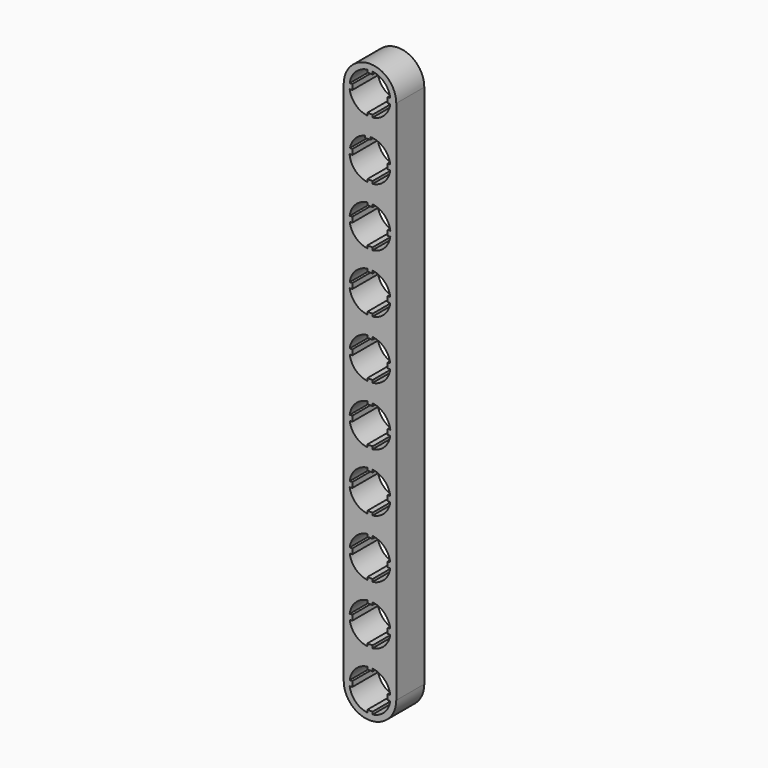
from build123d import *

# Parameters (mm, degrees)
F1_DEPTH = 7.62


# Not quite as in the source:
# - a feature names something its author has since deleted; it is built from what else it names


with BuildPart() as f1:
    # F0 (on Front) → F1 (new body)
    with BuildSketch(Plane.XZ):
        with BuildLine():
            ThreePointArc((-5.715, 47.4482442445), (0, 41.7332442445), (5.715, 47.4482442445))
            ThreePointArc((5.715, 47.4482442445), (0, 53.1632442445), (-5.715, 47.4482442445))
        make_face()
        with BuildLine():
            ThreePointArc((4.4081076155, 48.0197442445), (4.4357673153, 47.7345890096), (4.445, 47.4482442445))
            ThreePointArc((4.445, 47.4482442445), (4.4357673153, 47.1618994794), (4.4081076155, 46.8767442445))
            ThreePointArc((4.4081076155, 46.8767442445), (3.1430896424, 44.3051546021), (0.5715, 43.040136629))
            ThreePointArc((0.5715, 43.040136629), (0, 43.0032442445), (-0.5715, 43.040136629))
            ThreePointArc((-0.5715, 43.040136629), (-3.1430896424, 44.3051546021), (-4.4081076155, 46.8767442445))
            ThreePointArc((-4.4081076155, 46.8767442445), (-4.445, 47.4482442445), (-4.4081076155, 48.0197442445))
            ThreePointArc((-4.4081076155, 48.0197442445), (-3.1430896424, 50.5913338869), (-0.5715, 51.85635186))
            ThreePointArc((-0.5715, 51.85635186), (0, 51.8932442445), (0.5715, 51.85635186))
            ThreePointArc((0.5715, 51.85635186), (3.1430896424, 50.5913338869), (4.4081076155, 48.0197442445))
        make_face(mode=Mode.SUBTRACT)
        with BuildLine():
            Line((5.715, 34.7482442445), (5.715, 47.4482442445))
            ThreePointArc((5.715, 47.4482442445), (0, 41.7332442445), (-5.715, 47.4482442445))
            Line((-5.715, 47.4482442445), (-5.715, 34.7482442445))
            ThreePointArc((-5.715, 34.7482442445), (0, 40.4632442445), (5.715, 34.7482442445))
        make_face()
        with BuildLine():
            ThreePointArc((-5.715, 34.7482442445), (0, 29.0332442445), (5.715, 34.7482442445))
            ThreePointArc((5.715, 34.7482442445), (0, 40.4632442445), (-5.715, 34.7482442445))
        make_face()
        with BuildLine():
            ThreePointArc((4.4081076155, 35.3197442445), (4.4357673153, 35.0345890096), (4.445, 34.7482442445))
            ThreePointArc((4.445, 34.7482442445), (4.4357673153, 34.4618994794), (4.4081076155, 34.1767442445))
            ThreePointArc((4.4081076155, 34.1767442445), (3.1430896424, 31.6051546021), (0.5715, 30.340136629))
            ThreePointArc((0.5715, 30.340136629), (0, 30.3032442445), (-0.5715, 30.340136629))
            ThreePointArc((-0.5715, 30.340136629), (-3.2458434243, 31.7113831241), (-4.4363415477, 34.4709381461))
            ThreePointArc((-4.4363415477, 34.4709381461), (-4.4350889005, 35.0449114731), (-4.3598852128, 35.6139381461))
            ThreePointArc((-4.3598852128, 35.6139381461), (-3.2117417195, 37.821148429), (-1.0573885644, 39.0656455953))
            ThreePointArc((-1.0573885644, 39.0656455953), (-0.4900057315, 39.1661531823), (0.0856114356, 39.1924197228))
            ThreePointArc((0.0856114356, 39.1924197228), (2.9661054546, 38.0588700814), (4.4081076155, 35.3197442445))
        make_face(mode=Mode.SUBTRACT)
        with BuildLine():
            Line((5.715, 22.0482442445), (5.715, 34.7482442445))
            ThreePointArc((5.715, 34.7482442445), (0, 29.0332442445), (-5.715, 34.7482442445))
            Line((-5.715, 34.7482442445), (-5.715, 22.0482442445))
            ThreePointArc((-5.715, 22.0482442445), (0, 27.7632442445), (5.715, 22.0482442445))
        make_face()
        with BuildLine():
            ThreePointArc((-5.715, 22.0482442445), (0, 16.3332442445), (5.715, 22.0482442445))
            ThreePointArc((5.715, 22.0482442445), (0, 27.7632442445), (-5.715, 22.0482442445))
        make_face()
        with BuildLine():
            ThreePointArc((4.4081076155, 22.6197442445), (4.4357673153, 22.3345890096), (4.445, 22.0482442445))
            ThreePointArc((4.445, 22.0482442445), (4.4357673153, 21.7618994794), (4.4081076155, 21.4767442445))
            ThreePointArc((4.4081076155, 21.4767442445), (3.1430896424, 18.9051546021), (0.5715, 17.640136629))
            ThreePointArc((0.5715, 17.640136629), (0, 17.6032442445), (-0.5715, 17.640136629))
            ThreePointArc((-0.5715, 17.640136629), (-3.1430896424, 18.9051546021), (-4.4081076155, 21.4767442445))
            ThreePointArc((-4.4081076155, 21.4767442445), (-4.445, 22.0482442445), (-4.4081076155, 22.6197442445))
            ThreePointArc((-4.4081076155, 22.6197442445), (-3.1430896424, 25.1913338869), (-0.5715, 26.45635186))
            ThreePointArc((-0.5715, 26.45635186), (0, 26.4932442445), (0.5715, 26.45635186))
            ThreePointArc((0.5715, 26.45635186), (3.1430896424, 25.1913338869), (4.4081076155, 22.6197442445))
        make_face(mode=Mode.SUBTRACT)
        with BuildLine():
            Line((5.715, 9.3482442445), (5.715, 22.0482442445))
            ThreePointArc((5.715, 22.0482442445), (0, 16.3332442445), (-5.715, 22.0482442445))
            Line((-5.715, 22.0482442445), (-5.715, 9.348244273))
            ThreePointArc((-5.715, 9.348244273), (1.42e-08, 15.0632442445), (5.715, 9.3482442445))
        make_face()
        with BuildLine():
            ThreePointArc((-5.715, 9.348244273), (-1.42e-08, 3.6332442445), (5.715, 9.3482442445))
            ThreePointArc((5.715, 9.3482442445), (1.42e-08, 15.0632442445), (-5.715, 9.348244273))
        make_face()
        with BuildLine():
            ThreePointArc((4.4081076155, 9.9197442445), (4.4357673153, 9.6345890096), (4.445, 9.3482442445))
            ThreePointArc((4.445, 9.3482442445), (4.4357673153, 9.0618994794), (4.4081076155, 8.7767442445))
            ThreePointArc((4.4081076155, 8.7767442445), (3.1430896424, 6.2051546021), (0.5715, 4.940136629))
            ThreePointArc((0.5715, 4.940136629), (0, 4.9032442445), (-0.5715, 4.940136629))
            ThreePointArc((-0.5715, 4.940136629), (-3.1430896424, 6.2051546021), (-4.4081076155, 8.7767442445))
            ThreePointArc((-4.4081076155, 8.7767442445), (-4.445, 9.3482442445), (-4.4081076155, 9.9197442445))
            ThreePointArc((-4.4081076155, 9.9197442445), (-3.1430896424, 12.4913338869), (-0.5715, 13.75635186))
            ThreePointArc((-0.5715, 13.75635186), (0, 13.7932442445), (0.5715, 13.75635186))
            ThreePointArc((0.5715, 13.75635186), (3.1430896424, 12.4913338869), (4.4081076155, 9.9197442445))
        make_face(mode=Mode.SUBTRACT)
        with BuildLine():
            Line((5.715, -3.3517557555), (5.715, 9.3482442445))
            ThreePointArc((5.715, 9.3482442445), (-1.42e-08, 3.6332442445), (-5.715, 9.348244273))
            Line((-5.715, 9.348244273), (-5.715, -3.3517557536))
            ThreePointArc((-5.715, -3.3517557536), (9e-10, 2.3632442445), (5.715, -3.3517557555))
        make_face()
        with BuildLine():
            ThreePointArc((-5.715, -3.3517557536), (-9e-10, -9.0667557555), (5.715, -3.3517557555))
            ThreePointArc((5.715, -3.3517557555), (9e-10, 2.3632442445), (-5.715, -3.3517557536))
        make_face()
        with BuildLine():
            ThreePointArc((4.4081076155, -2.7802557555), (4.4357673153, -3.0654109904), (4.445, -3.3517557555))
            ThreePointArc((4.445, -3.3517557555), (4.4357673153, -3.6381005206), (4.4081076155, -3.9232557555))
            ThreePointArc((4.4081076155, -3.9232557555), (3.1430896424, -6.4948453979), (0.5715, -7.759863371))
            ThreePointArc((0.5715, -7.759863371), (0, -7.7967557555), (-0.5715, -7.759863371))
            ThreePointArc((-0.5715, -7.759863371), (-3.1430896424, -6.4948453979), (-4.4081076155, -3.9232557555))
            ThreePointArc((-4.4081076155, -3.9232557555), (-4.445, -3.3517557555), (-4.4081076155, -2.7802557555))
            ThreePointArc((-4.4081076155, -2.7802557555), (-3.1430896424, -0.2086661131), (-0.5715, 1.05635186))
            ThreePointArc((-0.5715, 1.05635186), (0, 1.0932442445), (0.5715, 1.05635186))
            ThreePointArc((0.5715, 1.05635186), (3.1430896424, -0.2086661131), (4.4081076155, -2.7802557555))
        make_face(mode=Mode.SUBTRACT)
        with BuildLine():
            Line((5.715, -16.0517557555), (5.715, -3.3517557555))
            ThreePointArc((5.715, -3.3517557555), (-9e-10, -9.0667557555), (-5.715, -3.3517557536))
            Line((-5.715, -3.3517557536), (-5.715, -16.0517557555))
            ThreePointArc((-5.715, -16.0517557555), (0, -10.3367557555), (5.715, -16.0517557555))
        make_face()
        with BuildLine():
            ThreePointArc((-5.715, -16.0517557555), (0, -21.7667557555), (5.715, -16.0517557555))
            ThreePointArc((5.715, -16.0517557555), (0, -10.3367557555), (-5.715, -16.0517557555))
        make_face()
        with BuildLine():
            ThreePointArc((4.4081076155, -15.4802557555), (4.4357673153, -15.7654109904), (4.445, -16.0517557555))
            ThreePointArc((4.445, -16.0517557555), (4.4357673153, -16.3381005206), (4.4081076155, -16.6232557555))
            ThreePointArc((4.4081076155, -16.6232557555), (3.1430896424, -19.1948453979), (0.5715, -20.459863371))
            ThreePointArc((0.5715, -20.459863371), (0, -20.4967557555), (-0.5715, -20.459863371))
            ThreePointArc((-0.5715, -20.459863371), (-3.1430896424, -19.1948453979), (-4.4081076155, -16.6232557555))
            ThreePointArc((-4.4081076155, -16.6232557555), (-4.445, -16.0517557555), (-4.4081076155, -15.4802557555))
            ThreePointArc((-4.4081076155, -15.4802557555), (-3.1430896424, -12.9086661131), (-0.5715, -11.64364814))
            ThreePointArc((-0.5715, -11.64364814), (0, -11.6067557555), (0.5715, -11.64364814))
            ThreePointArc((0.5715, -11.64364814), (3.1430896424, -12.9086661131), (4.4081076155, -15.4802557555))
        make_face(mode=Mode.SUBTRACT)
        with BuildLine():
            Line((5.715, -28.7517557555), (5.715, -16.0517557555))
            ThreePointArc((5.715, -16.0517557555), (0, -21.7667557555), (-5.715, -16.0517557555))
            Line((-5.715, -16.0517557555), (-5.715, -28.7517557555))
            ThreePointArc((-5.715, -28.7517557555), (0, -23.0367557555), (5.715, -28.7517557555))
        make_face()
        with BuildLine():
            ThreePointArc((-5.715, -28.7517557555), (0, -34.4667557555), (5.715, -28.7517557555))
            ThreePointArc((5.715, -28.7517557555), (0, -23.0367557555), (-5.715, -28.7517557555))
        make_face()
        with BuildLine():
            ThreePointArc((4.4081076155, -28.1802557555), (4.4357673153, -28.4654109904), (4.445, -28.7517557555))
            ThreePointArc((4.445, -28.7517557555), (4.4357673153, -29.0381005206), (4.4081076155, -29.3232557555))
            ThreePointArc((4.4081076155, -29.3232557555), (3.1430896424, -31.8948453979), (0.5715, -33.159863371))
            ThreePointArc((0.5715, -33.159863371), (0, -33.1967557555), (-0.5715, -33.159863371))
            ThreePointArc((-0.5715, -33.159863371), (-3.1430896424, -31.8948453979), (-4.4081076155, -29.3232557555))
            ThreePointArc((-4.4081076155, -29.3232557555), (-4.445, -28.7517557555), (-4.4081076155, -28.1802557555))
            ThreePointArc((-4.4081076155, -28.1802557555), (-3.1430896424, -25.6086661131), (-0.5715, -24.34364814))
            ThreePointArc((-0.5715, -24.34364814), (0, -24.3067557555), (0.5715, -24.34364814))
            ThreePointArc((0.5715, -24.34364814), (3.1430896424, -25.6086661131), (4.4081076155, -28.1802557555))
        make_face(mode=Mode.SUBTRACT)
        with BuildLine():
            Line((5.715, -41.4517557555), (5.715, -28.7517557555))
            ThreePointArc((5.715, -28.7517557555), (0, -34.4667557555), (-5.715, -28.7517557555))
            Line((-5.715, -28.7517557555), (-5.715, -41.4517557757))
            ThreePointArc((-5.715, -41.4517557757), (-1.01e-08, -35.7367557555), (5.715, -41.4517557555))
        make_face()
        with BuildLine():
            ThreePointArc((-5.715, -41.4517557757), (1.01e-08, -47.1667557555), (5.715, -41.4517557555))
            ThreePointArc((5.715, -41.4517557555), (-1.01e-08, -35.7367557555), (-5.715, -41.4517557757))
        make_face()
        with BuildLine():
            ThreePointArc((4.4081076155, -40.8802557555), (4.4357673153, -41.1654109904), (4.445, -41.4517557555))
            ThreePointArc((4.445, -41.4517557555), (4.4357673153, -41.7381005206), (4.4081076155, -42.0232557555))
            ThreePointArc((4.4081076155, -42.0232557555), (3.1430896424, -44.5948453979), (0.5715, -45.859863371))
            ThreePointArc((0.5715, -45.859863371), (0, -45.8967557555), (-0.5715, -45.859863371))
            ThreePointArc((-0.5715, -45.859863371), (-3.1430896424, -44.5948453979), (-4.4081076155, -42.0232557555))
            ThreePointArc((-4.4081076155, -42.0232557555), (-4.445, -41.4517557555), (-4.4081076155, -40.8802557555))
            ThreePointArc((-4.4081076155, -40.8802557555), (-3.1430896424, -38.3086661131), (-0.5715, -37.04364814))
            ThreePointArc((-0.5715, -37.04364814), (0, -37.0067557555), (0.5715, -37.04364814))
            ThreePointArc((0.5715, -37.04364814), (3.1430896424, -38.3086661131), (4.4081076155, -40.8802557555))
        make_face(mode=Mode.SUBTRACT)
        with BuildLine():
            Line((5.715, -54.1517557555), (5.715, -41.4517557555))
            ThreePointArc((5.715, -41.4517557555), (1.01e-08, -47.1667557555), (-5.715, -41.4517557757))
            Line((-5.715, -41.4517557757), (-5.715, -54.1517557757))
            ThreePointArc((-5.715, -54.1517557757), (-1.01e-08, -48.4367557555), (5.715, -54.1517557555))
        make_face()
        with BuildLine():
            ThreePointArc((-5.715, -54.1517557757), (1.01e-08, -59.8667557555), (5.715, -54.1517557555))
            ThreePointArc((5.715, -54.1517557555), (-1.01e-08, -48.4367557555), (-5.715, -54.1517557757))
        make_face()
        with BuildLine():
            ThreePointArc((4.4081076155, -53.5802557555), (4.4357673153, -53.8654109904), (4.445, -54.1517557555))
            ThreePointArc((4.445, -54.1517557555), (4.4357673153, -54.4381005206), (4.4081076155, -54.7232557555))
            ThreePointArc((4.4081076155, -54.7232557555), (3.1430896424, -57.2948453979), (0.5715, -58.559863371))
            ThreePointArc((0.5715, -58.559863371), (0, -58.5967557555), (-0.5715, -58.559863371))
            ThreePointArc((-0.5715, -58.559863371), (-3.1430896424, -57.2948453979), (-4.4081076155, -54.7232557555))
            ThreePointArc((-4.4081076155, -54.7232557555), (-4.445, -54.1517557555), (-4.4081076155, -53.5802557555))
            ThreePointArc((-4.4081076155, -53.5802557555), (-3.1430896424, -51.0086661131), (-0.5715, -49.74364814))
            ThreePointArc((-0.5715, -49.74364814), (0, -49.7067557555), (0.5715, -49.74364814))
            ThreePointArc((0.5715, -49.74364814), (3.1430896424, -51.0086661131), (4.4081076155, -53.5802557555))
        make_face(mode=Mode.SUBTRACT)
        with BuildLine():
            Line((5.715, -66.8517557555), (5.715, -54.1517557555))
            ThreePointArc((5.715, -54.1517557555), (1.01e-08, -59.8667557555), (-5.715, -54.1517557757))
            Line((-5.715, -54.1517557757), (-5.715, -66.8517557555))
            ThreePointArc((-5.715, -66.8517557555), (0, -61.1367557555), (5.715, -66.8517557555))
        make_face()
        with BuildLine():
            ThreePointArc((-5.715, -66.8517557555), (0, -72.5667557555), (5.715, -66.8517557555))
            ThreePointArc((5.715, -66.8517557555), (0, -61.1367557555), (-5.715, -66.8517557555))
        make_face()
        with BuildLine():
            ThreePointArc((4.4081076155, -66.2802557555), (4.4357673153, -66.5654109904), (4.445, -66.8517557555))
            ThreePointArc((4.445, -66.8517557555), (4.4357673153, -67.1381005206), (4.4081076155, -67.4232557555))
            ThreePointArc((4.4081076155, -67.4232557555), (3.1430896424, -69.9948453979), (0.5715, -71.259863371))
            ThreePointArc((0.5715, -71.259863371), (0, -71.2967557555), (-0.5715, -71.259863371))
            ThreePointArc((-0.5715, -71.259863371), (-3.1430896424, -69.9948453979), (-4.4081076155, -67.4232557555))
            ThreePointArc((-4.4081076155, -67.4232557555), (-4.445, -66.8517557555), (-4.4081076155, -66.2802557555))
            ThreePointArc((-4.4081076155, -66.2802557555), (-3.1430896424, -63.7086661131), (-0.5715, -62.44364814))
            ThreePointArc((-0.5715, -62.44364814), (0, -62.4067557555), (0.5715, -62.44364814))
            ThreePointArc((0.5715, -62.44364814), (3.1430896424, -63.7086661131), (4.4081076155, -66.2802557555))
        make_face(mode=Mode.SUBTRACT)
        with BuildLine():
            Line((0.5715, 51.29755186), (0.5715, 51.85635186))
            ThreePointArc((0.5715, 51.85635186), (0, 51.8932442445), (-0.5715, 51.85635186))
            Line((-0.5715, 51.85635186), (-0.5715, 51.29755186))
            Line((-0.5715, 51.29755186), (0.5715, 51.29755186))
        make_face()
        with BuildLine():
            ThreePointArc((4.4081076155, 46.8767442445), (4.4357673153, 47.1618994794), (4.445, 47.4482442445))
            ThreePointArc((4.445, 47.4482442445), (4.4357673153, 47.7345890096), (4.4081076155, 48.0197442445))
            Line((4.4081076155, 48.0197442445), (3.8493076155, 48.0197442445))
            Line((3.8493076155, 48.0197442445), (3.8493076155, 46.8767442445))
            Line((3.8493076155, 46.8767442445), (4.4081076155, 46.8767442445))
        make_face()
        with BuildLine():
            ThreePointArc((-0.5715, 43.040136629), (0, 43.0032442445), (0.5715, 43.040136629))
            Line((0.5715, 43.040136629), (0.5715, 43.598936629))
            Line((0.5715, 43.598936629), (-0.5715, 43.598936629))
            Line((-0.5715, 43.598936629), (-0.5715, 43.040136629))
        make_face()
        with BuildLine():
            Line((-3.8493076155, 48.0197442445), (-4.4081076155, 48.0197442445))
            ThreePointArc((-4.4081076155, 48.0197442445), (-4.445, 47.4482442445), (-4.4081076155, 46.8767442445))
            Line((-4.4081076155, 46.8767442445), (-3.8493076155, 46.8767442445))
            Line((-3.8493076155, 46.8767442445), (-3.8493076155, 48.0197442445))
        make_face()
        with BuildLine():
            ThreePointArc((4.4081076155, -67.4232557555), (4.4357673153, -67.1381005206), (4.445, -66.8517557555))
            ThreePointArc((4.445, -66.8517557555), (4.4357673153, -66.5654109904), (4.4081076155, -66.2802557555))
            Line((4.4081076155, -66.2802557555), (3.8493076155, -66.2802557555))
            Line((3.8493076155, -66.2802557555), (3.8493076155, -67.4232557555))
            Line((3.8493076155, -67.4232557555), (4.4081076155, -67.4232557555))
        make_face()
        with BuildLine():
            ThreePointArc((4.4081076155, 8.7767442445), (4.4357673153, 9.0618994794), (4.445, 9.3482442445))
            ThreePointArc((4.445, 9.3482442445), (4.4357673153, 9.6345890096), (4.4081076155, 9.9197442445))
            Line((4.4081076155, 9.9197442445), (3.8493076155, 9.9197442445))
            Line((3.8493076155, 9.9197442445), (3.8493076155, 8.7767442445))
            Line((3.8493076155, 8.7767442445), (4.4081076155, 8.7767442445))
        make_face()
        with BuildLine():
            Line((-3.8493076155, -15.4802557555), (-4.4081076155, -15.4802557555))
            ThreePointArc((-4.4081076155, -15.4802557555), (-4.445, -16.0517557555), (-4.4081076155, -16.6232557555))
            Line((-4.4081076155, -16.6232557555), (-3.8493076155, -16.6232557555))
            Line((-3.8493076155, -16.6232557555), (-3.8493076155, -15.4802557555))
        make_face()
        with BuildLine():
            Line((0.0856114356, 38.6336197228), (0.0856114356, 39.1924197228))
            ThreePointArc((0.0856114356, 39.1924197228), (-0.4900057315, 39.1661531823), (-1.0573885644, 39.0656455953))
            Line((-1.0573885644, 39.0656455953), (-1.0573885644, 38.6336197228))
            Line((-1.0573885644, 38.6336197228), (0.0856114356, 38.6336197228))
        make_face()
        with BuildLine():
            Line((-3.8010852128, 35.6139381461), (-4.3598852128, 35.6139381461))
            ThreePointArc((-4.3598852128, 35.6139381461), (-4.4350889005, 35.0449114731), (-4.4363415477, 34.4709381461))
            Line((-4.4363415477, 34.4709381461), (-3.8010852128, 34.4709381461))
            Line((-3.8010852128, 34.4709381461), (-3.8010852128, 35.6139381461))
        make_face()
        with BuildLine():
            ThreePointArc((-0.5715, 30.340136629), (0, 30.3032442445), (0.5715, 30.340136629))
            Line((0.5715, 30.340136629), (0.5715, 30.898936629))
            Line((0.5715, 30.898936629), (-0.5715, 30.898936629))
            Line((-0.5715, 30.898936629), (-0.5715, 30.340136629))
        make_face()
        with BuildLine():
            ThreePointArc((4.4081076155, 34.1767442445), (4.4357673153, 34.4618994794), (4.445, 34.7482442445))
            ThreePointArc((4.445, 34.7482442445), (4.4357673153, 35.0345890096), (4.4081076155, 35.3197442445))
            Line((4.4081076155, 35.3197442445), (3.8493076155, 35.3197442445))
            Line((3.8493076155, 35.3197442445), (3.8493076155, 34.1767442445))
            Line((3.8493076155, 34.1767442445), (4.4081076155, 34.1767442445))
        make_face()
        with BuildLine():
            Line((0.5715, 25.89755186), (0.5715, 26.45635186))
            ThreePointArc((0.5715, 26.45635186), (0, 26.4932442445), (-0.5715, 26.45635186))
            Line((-0.5715, 26.45635186), (-0.5715, 25.89755186))
            Line((-0.5715, 25.89755186), (0.5715, 25.89755186))
        make_face()
        with BuildLine():
            Line((-3.8493076155, 22.6197442445), (-4.4081076155, 22.6197442445))
            ThreePointArc((-4.4081076155, 22.6197442445), (-4.445, 22.0482442445), (-4.4081076155, 21.4767442445))
            Line((-4.4081076155, 21.4767442445), (-3.8493076155, 21.4767442445))
            Line((-3.8493076155, 21.4767442445), (-3.8493076155, 22.6197442445))
        make_face()
        with BuildLine():
            ThreePointArc((4.4081076155, 21.4767442445), (4.4357673153, 21.7618994794), (4.445, 22.0482442445))
            ThreePointArc((4.445, 22.0482442445), (4.4357673153, 22.3345890096), (4.4081076155, 22.6197442445))
            Line((4.4081076155, 22.6197442445), (3.8493076155, 22.6197442445))
            Line((3.8493076155, 22.6197442445), (3.8493076155, 21.4767442445))
            Line((3.8493076155, 21.4767442445), (4.4081076155, 21.4767442445))
        make_face()
        with BuildLine():
            ThreePointArc((-0.5715, 17.640136629), (0, 17.6032442445), (0.5715, 17.640136629))
            Line((0.5715, 17.640136629), (0.5715, 18.198936629))
            Line((0.5715, 18.198936629), (-0.5715, 18.198936629))
            Line((-0.5715, 18.198936629), (-0.5715, 17.640136629))
        make_face()
        with BuildLine():
            Line((0.5715, 13.19755186), (0.5715, 13.75635186))
            ThreePointArc((0.5715, 13.75635186), (0, 13.7932442445), (-0.5715, 13.75635186))
            Line((-0.5715, 13.75635186), (-0.5715, 13.19755186))
            Line((-0.5715, 13.19755186), (0.5715, 13.19755186))
        make_face()
        with BuildLine():
            Line((-3.8493076155, 9.9197442445), (-4.4081076155, 9.9197442445))
            ThreePointArc((-4.4081076155, 9.9197442445), (-4.445, 9.3482442445), (-4.4081076155, 8.7767442445))
            Line((-4.4081076155, 8.7767442445), (-3.8493076155, 8.7767442445))
            Line((-3.8493076155, 8.7767442445), (-3.8493076155, 9.9197442445))
        make_face()
        with BuildLine():
            ThreePointArc((-0.5715, 4.940136629), (0, 4.9032442445), (0.5715, 4.940136629))
            Line((0.5715, 4.940136629), (0.5715, 5.498936629))
            Line((0.5715, 5.498936629), (-0.5715, 5.498936629))
            Line((-0.5715, 5.498936629), (-0.5715, 4.940136629))
        make_face()
        with BuildLine():
            Line((0.5715, 0.49755186), (0.5715, 1.05635186))
            ThreePointArc((0.5715, 1.05635186), (0, 1.0932442445), (-0.5715, 1.05635186))
            Line((-0.5715, 1.05635186), (-0.5715, 0.49755186))
            Line((-0.5715, 0.49755186), (0.5715, 0.49755186))
        make_face()
        with BuildLine():
            ThreePointArc((4.4081076155, -3.9232557555), (4.4357673153, -3.6381005206), (4.445, -3.3517557555))
            ThreePointArc((4.445, -3.3517557555), (4.4357673153, -3.0654109904), (4.4081076155, -2.7802557555))
            Line((4.4081076155, -2.7802557555), (3.8493076155, -2.7802557555))
            Line((3.8493076155, -2.7802557555), (3.8493076155, -3.9232557555))
            Line((3.8493076155, -3.9232557555), (4.4081076155, -3.9232557555))
        make_face()
        with BuildLine():
            ThreePointArc((-0.5715, -7.759863371), (0, -7.7967557555), (0.5715, -7.759863371))
            Line((0.5715, -7.759863371), (0.5715, -7.201063371))
            Line((0.5715, -7.201063371), (-0.5715, -7.201063371))
            Line((-0.5715, -7.201063371), (-0.5715, -7.759863371))
        make_face()
        with BuildLine():
            Line((-3.8493076155, -2.7802557555), (-4.4081076155, -2.7802557555))
            ThreePointArc((-4.4081076155, -2.7802557555), (-4.445, -3.3517557555), (-4.4081076155, -3.9232557555))
            Line((-4.4081076155, -3.9232557555), (-3.8493076155, -3.9232557555))
            Line((-3.8493076155, -3.9232557555), (-3.8493076155, -2.7802557555))
        make_face()
        with BuildLine():
            Line((0.5715, -12.20244814), (0.5715, -11.64364814))
            ThreePointArc((0.5715, -11.64364814), (0, -11.6067557555), (-0.5715, -11.64364814))
            Line((-0.5715, -11.64364814), (-0.5715, -12.20244814))
            Line((-0.5715, -12.20244814), (0.5715, -12.20244814))
        make_face()
        with BuildLine():
            ThreePointArc((4.4081076155, -16.6232557555), (4.4357673153, -16.3381005206), (4.445, -16.0517557555))
            ThreePointArc((4.445, -16.0517557555), (4.4357673153, -15.7654109904), (4.4081076155, -15.4802557555))
            Line((4.4081076155, -15.4802557555), (3.8493076155, -15.4802557555))
            Line((3.8493076155, -15.4802557555), (3.8493076155, -16.6232557555))
            Line((3.8493076155, -16.6232557555), (4.4081076155, -16.6232557555))
        make_face()
        with BuildLine():
            ThreePointArc((-0.5715, -20.459863371), (0, -20.4967557555), (0.5715, -20.459863371))
            Line((0.5715, -20.459863371), (0.5715, -19.901063371))
            Line((0.5715, -19.901063371), (-0.5715, -19.901063371))
            Line((-0.5715, -19.901063371), (-0.5715, -20.459863371))
        make_face()
        with BuildLine():
            Line((0.5715, -24.90244814), (0.5715, -24.34364814))
            ThreePointArc((0.5715, -24.34364814), (0, -24.3067557555), (-0.5715, -24.34364814))
            Line((-0.5715, -24.34364814), (-0.5715, -24.90244814))
            Line((-0.5715, -24.90244814), (0.5715, -24.90244814))
        make_face()
        with BuildLine():
            ThreePointArc((4.4081076155, -29.3232557555), (4.4357673153, -29.0381005206), (4.445, -28.7517557555))
            ThreePointArc((4.445, -28.7517557555), (4.4357673153, -28.4654109904), (4.4081076155, -28.1802557555))
            Line((4.4081076155, -28.1802557555), (3.8493076155, -28.1802557555))
            Line((3.8493076155, -28.1802557555), (3.8493076155, -29.3232557555))
            Line((3.8493076155, -29.3232557555), (4.4081076155, -29.3232557555))
        make_face()
        with BuildLine():
            Line((-3.8493076155, -28.1802557555), (-4.4081076155, -28.1802557555))
            ThreePointArc((-4.4081076155, -28.1802557555), (-4.445, -28.7517557555), (-4.4081076155, -29.3232557555))
            Line((-4.4081076155, -29.3232557555), (-3.8493076155, -29.3232557555))
            Line((-3.8493076155, -29.3232557555), (-3.8493076155, -28.1802557555))
        make_face()
        with BuildLine():
            ThreePointArc((-0.5715, -33.159863371), (0, -33.1967557555), (0.5715, -33.159863371))
            Line((0.5715, -33.159863371), (0.5715, -32.601063371))
            Line((0.5715, -32.601063371), (-0.5715, -32.601063371))
            Line((-0.5715, -32.601063371), (-0.5715, -33.159863371))
        make_face()
        with BuildLine():
            Line((0.5715, -37.60244814), (0.5715, -37.04364814))
            ThreePointArc((0.5715, -37.04364814), (0, -37.0067557555), (-0.5715, -37.04364814))
            Line((-0.5715, -37.04364814), (-0.5715, -37.60244814))
            Line((-0.5715, -37.60244814), (0.5715, -37.60244814))
        make_face()
        with BuildLine():
            ThreePointArc((4.4081076155, -42.0232557555), (4.4357673153, -41.7381005206), (4.445, -41.4517557555))
            ThreePointArc((4.445, -41.4517557555), (4.4357673153, -41.1654109904), (4.4081076155, -40.8802557555))
            Line((4.4081076155, -40.8802557555), (3.8493076155, -40.8802557555))
            Line((3.8493076155, -40.8802557555), (3.8493076155, -42.0232557555))
            Line((3.8493076155, -42.0232557555), (4.4081076155, -42.0232557555))
        make_face()
        with BuildLine():
            Line((-3.8493076155, -40.8802557555), (-4.4081076155, -40.8802557555))
            ThreePointArc((-4.4081076155, -40.8802557555), (-4.445, -41.4517557555), (-4.4081076155, -42.0232557555))
            Line((-4.4081076155, -42.0232557555), (-3.8493076155, -42.0232557555))
            Line((-3.8493076155, -42.0232557555), (-3.8493076155, -40.8802557555))
        make_face()
        with BuildLine():
            ThreePointArc((-0.5715, -45.859863371), (0, -45.8967557555), (0.5715, -45.859863371))
            Line((0.5715, -45.859863371), (0.5715, -45.301063371))
            Line((0.5715, -45.301063371), (-0.5715, -45.301063371))
            Line((-0.5715, -45.301063371), (-0.5715, -45.859863371))
        make_face()
        with BuildLine():
            Line((0.5715, -50.30244814), (0.5715, -49.74364814))
            ThreePointArc((0.5715, -49.74364814), (0, -49.7067557555), (-0.5715, -49.74364814))
            Line((-0.5715, -49.74364814), (-0.5715, -50.30244814))
            Line((-0.5715, -50.30244814), (0.5715, -50.30244814))
        make_face()
        with BuildLine():
            ThreePointArc((4.4081076155, -54.7232557555), (4.4357673153, -54.4381005206), (4.445, -54.1517557555))
            ThreePointArc((4.445, -54.1517557555), (4.4357673153, -53.8654109904), (4.4081076155, -53.5802557555))
            Line((4.4081076155, -53.5802557555), (3.8493076155, -53.5802557555))
            Line((3.8493076155, -53.5802557555), (3.8493076155, -54.7232557555))
            Line((3.8493076155, -54.7232557555), (4.4081076155, -54.7232557555))
        make_face()
        with BuildLine():
            ThreePointArc((-0.5715, -58.559863371), (0, -58.5967557555), (0.5715, -58.559863371))
            Line((0.5715, -58.559863371), (0.5715, -58.001063371))
            Line((0.5715, -58.001063371), (-0.5715, -58.001063371))
            Line((-0.5715, -58.001063371), (-0.5715, -58.559863371))
        make_face()
        with BuildLine():
            Line((-3.8493076155, -53.5802557555), (-4.4081076155, -53.5802557555))
            ThreePointArc((-4.4081076155, -53.5802557555), (-4.445, -54.1517557555), (-4.4081076155, -54.7232557555))
            Line((-4.4081076155, -54.7232557555), (-3.8493076155, -54.7232557555))
            Line((-3.8493076155, -54.7232557555), (-3.8493076155, -53.5802557555))
        make_face()
        with BuildLine():
            Line((0.5715, -63.00244814), (0.5715, -62.44364814))
            ThreePointArc((0.5715, -62.44364814), (0, -62.4067557555), (-0.5715, -62.44364814))
            Line((-0.5715, -62.44364814), (-0.5715, -63.00244814))
            Line((-0.5715, -63.00244814), (0.5715, -63.00244814))
        make_face()
        with BuildLine():
            Line((-3.8493076155, -66.2802557555), (-4.4081076155, -66.2802557555))
            ThreePointArc((-4.4081076155, -66.2802557555), (-4.445, -66.8517557555), (-4.4081076155, -67.4232557555))
            Line((-4.4081076155, -67.4232557555), (-3.8493076155, -67.4232557555))
            Line((-3.8493076155, -67.4232557555), (-3.8493076155, -66.2802557555))
        make_face()
        with BuildLine():
            ThreePointArc((-0.5715, -71.259863371), (0, -71.2967557555), (0.5715, -71.259863371))
            Line((0.5715, -71.259863371), (0.5715, -70.701063371))
            Line((0.5715, -70.701063371), (-0.5715, -70.701063371))
            Line((-0.5715, -70.701063371), (-0.5715, -71.259863371))
        make_face()
    extrude(amount=F1_DEPTH)


solid = f1.part
